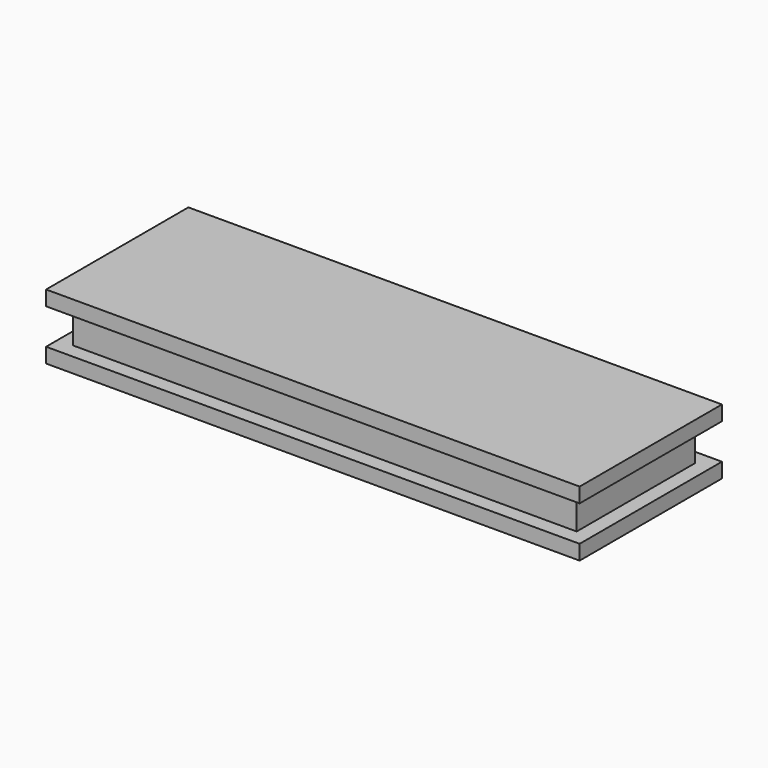
from build123d import *

# Parameters (mm, degrees)
F0_W     = 900
F0_H     = 300
F1_DEPTH = 25
F2_W     = 850
F2_H     = 250
F3_DEPTH = 60


# Not quite as in the source:
# - a pattern or mirror of a feature is missing from the dataset's text; its kind, count and spacing are read off the source's solid


with BuildPart() as f1:
    # F0 (on Top) → F1 (new body)
    with BuildSketch(Plane.XY):
        Rectangle(F0_W, F0_H)
    extrude(amount=F1_DEPTH)


with BuildPart() as f1_copies_1:
    # F1_copies: instance of F1
    add(f1.part.mirror(Plane.XY.offset(55)))


with BuildPart() as f1_1:
    add(f1.part)

    add(f1_copies_1.part)  # F3 merges F1_copies_1
    # F2 (on face) → F3 (join)
    with BuildSketch(Plane.XY.offset(25)):
        Rectangle(F2_W, F2_H)
    extrude(amount=F3_DEPTH)


solid = f1_1.part
